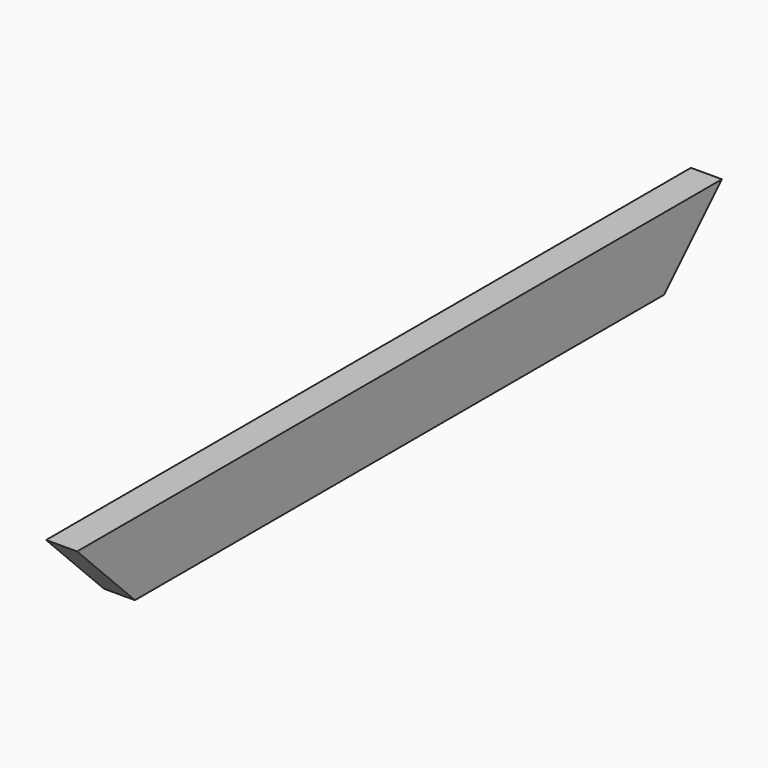
from build123d import *

# Parameters (mm, degrees)
F0_W     = 38.1
F0_H     = 88.9
F1_DEPTH = 495.3
F2_SIZE2 = 88.89999
F2_SIZE  = 88.89999
F3_SIZE2 = 88.89999
F3_SIZE  = 88.89999


# Not quite as in the source:
# - a fillet or chamfer is up to 0.001 mm smaller than in the source, because OpenCascade refuses the exact size


with BuildPart() as f1:
    # F0 (on Front) → F1 (new body, symmetric)
    with BuildSketch(Plane.XZ):
        Rectangle(F0_W, F0_H)
    extrude(amount=F1_DEPTH, both=True)

    # F2 (size 88.9 and 88.9 in the source; OpenCascade refuses exactly that, so slightly less here)
    f2_edges = [f1.edges().sort_by_distance(p)[0] for p in [
        (0, -495.3, -44.45),
    ]]
    chamfer(f2_edges, length=F2_SIZE, length2=F2_SIZE2)

    # F3 (size 88.9 and 88.9 in the source; OpenCascade refuses exactly that, so slightly less here)
    f3_edges = [f1.edges().sort_by_distance(p)[0] for p in [
        (0, 495.3, -44.45),
    ]]
    chamfer(f3_edges, length=F3_SIZE, length2=F3_SIZE2)


solid = f1.part
